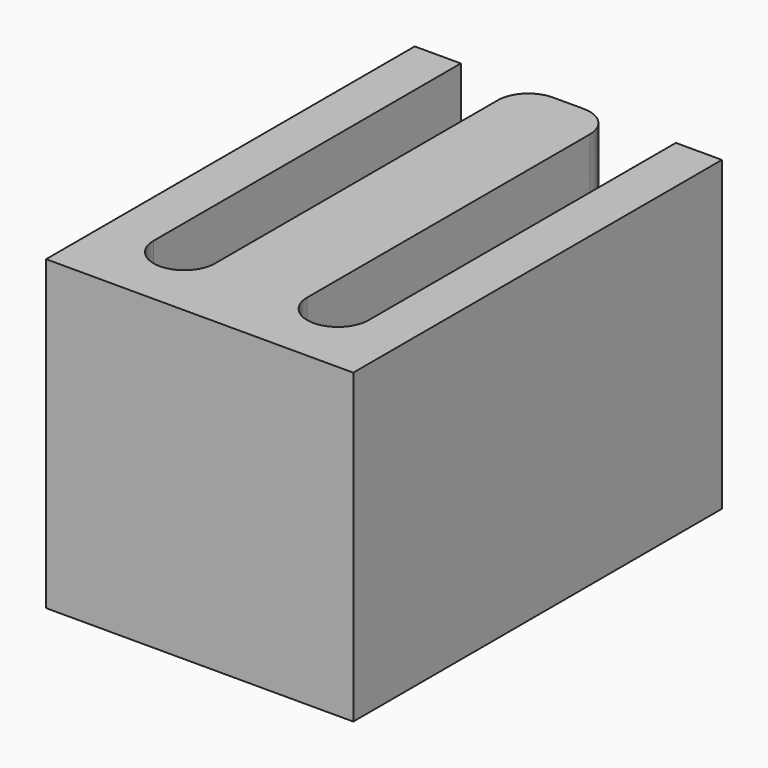
from build123d import *

# Parameters (mm, degrees)
F0_W     = 20
F0_H     = 30
F1_DEPTH = 20
F2_W     = 14
F2_H     = 27
F3_DEPTH = 15
F4_W     = 6
F4_H     = 10
F5_DEPTH = 27
F6_SIZE  = 5
F7_R     = 1.99999


# Not quite as in the source:
# - a fillet or chamfer is up to 0.001 mm smaller than in the source, because OpenCascade refuses the exact size


with BuildPart() as f1:
    # F0 (on Top) → F1 (new body)
    with BuildSketch(Plane.XY):
        with Locations((50, 60)):
            Rectangle(F0_W, F0_H)
    extrude(amount=F1_DEPTH)

    # F2 (on face) → F3 (cut)
    with BuildSketch(Plane.XY.offset(20)):
        with Locations((50, 61.5)):
            Rectangle(F2_W, F2_H)
    extrude(amount=-F3_DEPTH, mode=Mode.SUBTRACT)

    # F4 (on face) → F5 (join, through all)
    with BuildSketch(Plane(origin=(0, 48, 0), x_dir=(-1, 0, 0), z_dir=(0, 1, 0))):
        with Locations((-50, 15)):
            Rectangle(F4_W, F4_H)
    extrude(amount=F5_DEPTH)

    # F6
    f6_edges = [f1.edges().sort_by_distance(p)[0] for p in [
        (50, 75, 10),
    ]]
    chamfer(f6_edges, length=F6_SIZE)

    # F7 (radius 2 in the source; OpenCascade refuses exactly that, so slightly less here)
    f7_edges = [f1.edges().sort_by_distance(p)[0] for p in [
        (43, 48, 12.5),
        (47, 48, 15),
        (57, 48, 12.5),
        (53, 48, 15),
        (53, 75, 17.5),
        (47, 75, 17.5),
        (47, 72.5, 12.5),
        (53, 72.5, 12.5),
    ]]
    fillet(f7_edges, radius=F7_R)


solid = f1.part
